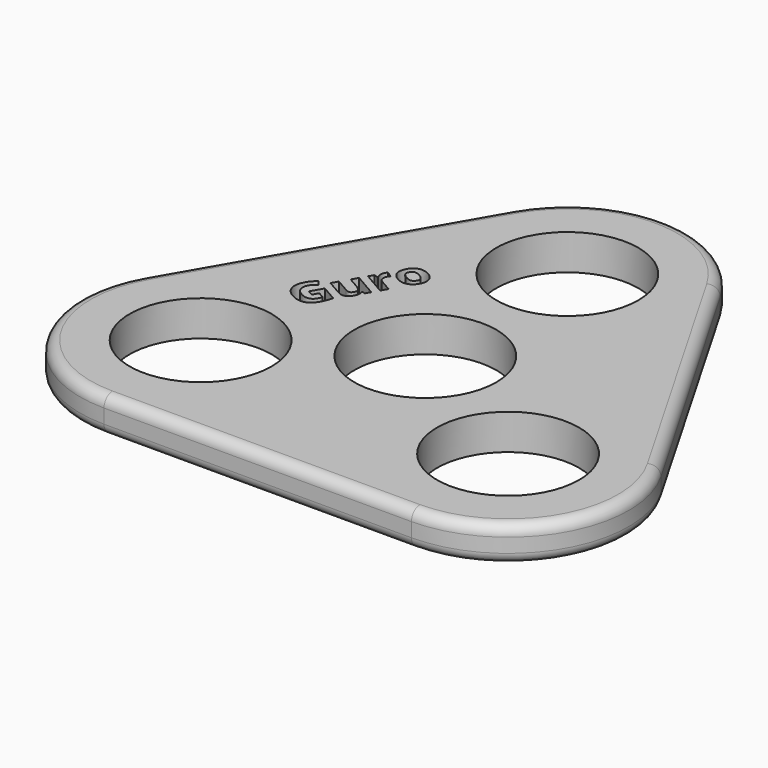
from build123d import *

# Parameters (mm, degrees)
F0_R         = 10
F1_DEPTH     = 5
F2_TEXT_SIZE = 6.7014176036
F3_DEPTH     = 5.001
F4_R         = 1.5


# Not quite as in the source:
# - Text() gives the source's letters only with a copy of the font that has no kerning and outlines rounded to 1/6400 em; it was checked with that copy


with BuildPart() as f1:
    # F0 (on Top) → F1 (new body)
    with BuildSketch(Plane.XY):
        with BuildLine():
            Line((36.366066065, -3.9878740959), (14.7224318643, 33.5))
            ThreePointArc((14.7224318643, 33.5), (0, 42), (-14.7224318643, 33.5))
            Line((-14.7224318643, 33.5), (-36.366066065, -3.9878740959))
            ThreePointArc((-36.366066065, -3.9878740959), (-36.366066065, -20.9878740959), (-21.6436342006, -29.4878740959))
            Line((-21.6436342006, -29.4878740959), (21.6436342006, -29.4878740959))
            ThreePointArc((21.6436342006, -29.4878740959), (36.366066065, -20.9878740959), (36.366066065, -3.9878740959))
        make_face()
        with Locations((-21.6436342006, -12.4878740959)):
            Circle(F0_R, mode=Mode.SUBTRACT)
        with BuildLine():
            ThreePointArc((9.9994813614, -0.1018454888), (-9.9998703395, 0.0509234047), (10, 0))
            ThreePointArc((10, 0), (9.9998703395, -0.0509234047), (9.9994813614, -0.1018454888))
        make_face(mode=Mode.SUBTRACT)
        with Locations((21.6436342006, -12.4878740959)):
            Circle(F0_R, mode=Mode.SUBTRACT)
        with Locations((0, 25)):
            Circle(F0_R, mode=Mode.SUBTRACT)
    extrude(amount=F1_DEPTH)

    # F2 (on face) → F3 (cut, through all)
    with BuildSketch(Plane.XY.offset(5)):
        with Locations(Location((-18.5011867434, 0.5914596841), (0, 0, 60))):
            Text('Guro', F2_TEXT_SIZE, font='Open Sans', font_style=FontStyle.BOLD, text_align=(TextAlign.LEFT, TextAlign.BOTTOM))
    extrude(amount=-F3_DEPTH, mode=Mode.SUBTRACT)

    # F4
    f4_edges = [f1.edges().sort_by_distance(p)[0] for p in [
        (-25.544249, 14.756063, 5),
        (0, -29.487874, 0),
        (-36.366066, -20.987874, 0),
    ]]
    fillet(f4_edges, radius=F4_R)


solid = f1.part
